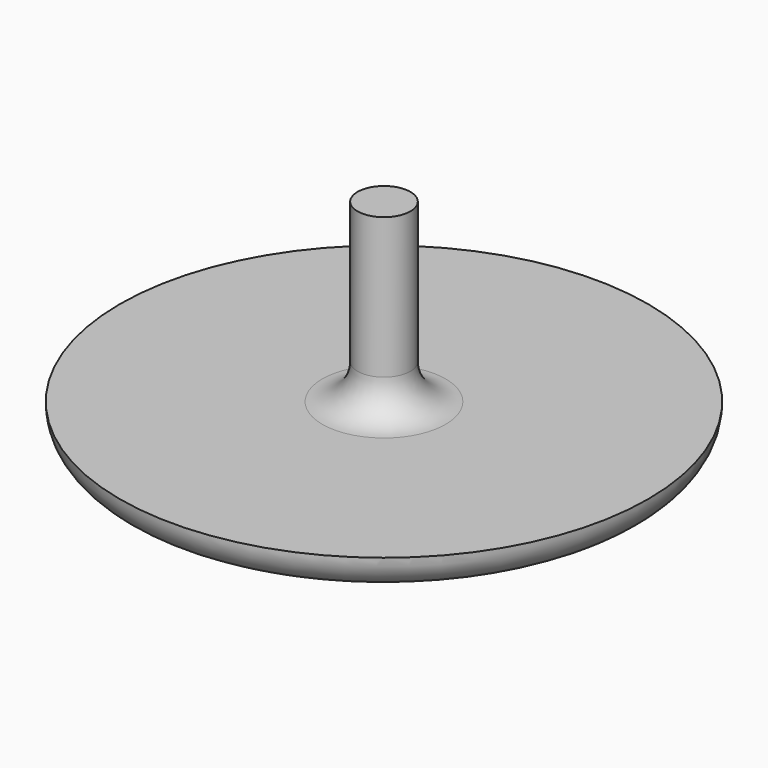
from build123d import *

# Parameters (mm, degrees)
F0_W = 1.5
F0_H = 10
F2_R = 1.99999


# Not quite as in the source:
# - a fillet or chamfer is up to 0.001 mm smaller than in the source, because OpenCascade refuses the exact size


with BuildPart() as f1:
    # F0 (on Front) → F1 (revolve)
    with BuildSketch(Plane.XZ):
        with Locations((-0.75, 7)):
            Rectangle(F0_W, F0_H)
        Polygon((-15, 0), (0, 0), (0, 2), (-1.5, 2), (-15, 2), align=None)
    revolve(axis=Axis((0, 0, 27.7387052774), (0, 0, 1)))

    # F2 (radius 2 in the source; OpenCascade refuses exactly that, so slightly less here)
    f2_edges = [f1.edges().sort_by_distance(p)[0] for p in [
        (15, 0, 0),
        (1.5, 0, 2),
    ]]
    fillet(f2_edges, radius=F2_R)


solid = f1.part
